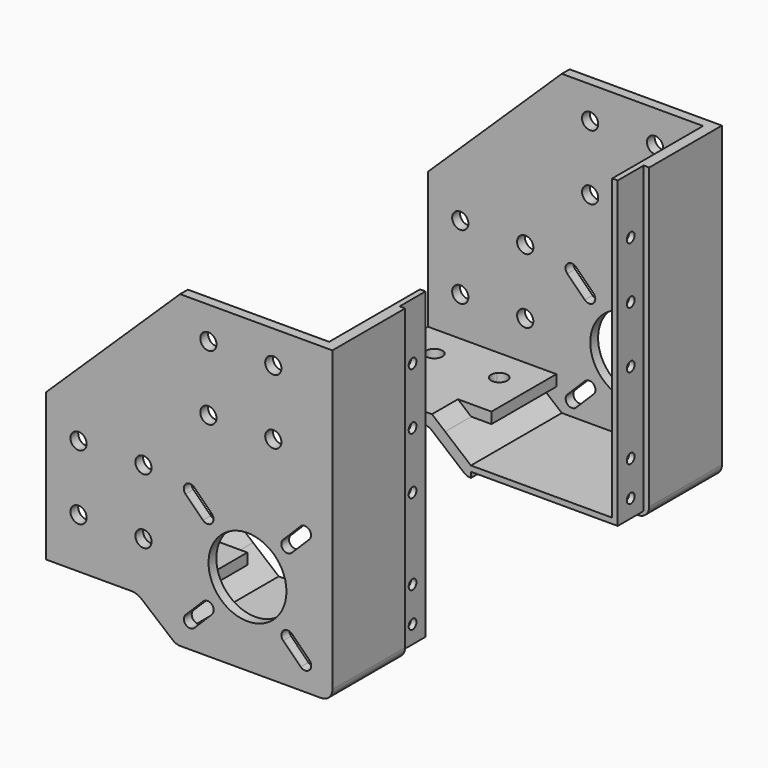
from build123d import *

# Parameters (mm, degrees)
F3_R         = 2.5
F3_R_2       = 12
F5_DEPTH     = 3
F6_DEPTH     = 28
F7_R         = 2.5
F8_DEPTH     = 12.5
F9_DEPTH     = 207
F11_DEPTH    = 10
F12_R        = 1.5
F13_DEPTH    = 1.7
F14_T1_DEPTH = 44.1548490014
F14_T3_DEPTH = 45
F15_R        = 5


# Not quite as in the source:
# - a fillet or chamfer that OpenCascade refuses, or shapes differently, is made with other operations: its cross-section is extruded or revolved along the edge and cut away or added
# - an extrude ends at something that could not be found from the text; its depth is read off the source's solid


with BuildPart() as f5:
    # F3 (on offset) → F5 (new body)
    with BuildSketch(Plane.XZ.offset(75)):
        Polygon((22.8, -22), (22.8, 22), (-11.1900709997, 22), (-20.7240998825, 30.0000001192), (-31.9999998808, 30.0000001192), (-61.9999998808, 30.0000001192), (-61.9999998808, -9.9999998808), (-61.9999998808, -11.9999998808), (-32.7240997633, -11.9999998808), (-20.7240998825, -22), align=None)
        with Locations((-51.9999998808, 1.192e-07)):
            Circle(F3_R, mode=Mode.SUBTRACT)
        with Locations((-31.9999998808, 1.192e-07)):
            Circle(F3_R, mode=Mode.SUBTRACT)
        with Locations((-51.9999998808, 20.0000001192)):
            Circle(F3_R, mode=Mode.SUBTRACT)
        with Locations((-31.9999998808, 20.0000001192)):
            Circle(F3_R, mode=Mode.SUBTRACT)
        with BuildLine():
            Line((-10.9146282961, -13.6954990502), (-16.2886398331, -19.0695105872))
            ThreePointArc((-16.2886398331, -19.0695105872), (-18.9756456016, -19.0695105872), (-18.9756456016, -16.3825048187))
            Line((-18.9756456016, -16.3825048187), (-13.6016340646, -11.0084932817))
            ThreePointArc((-13.6016340646, -11.0084932817), (-10.9146282961, -11.0084932817), (-10.9146282961, -13.6954990502))
        make_face(mode=Mode.SUBTRACT)
        with Locations((0.0469324928, 0.0079305583)):
            Circle(F3_R_2, mode=Mode.SUBTRACT)
        with BuildLine():
            Line((13.7503621014, -10.9536302305), (19.1243736384, -16.3276417676))
            ThreePointArc((19.1243736384, -16.3276417676), (19.1243736384, -19.0146475361), (16.4373678699, -19.0146475361))
            Line((16.4373678699, -19.0146475361), (11.0633563329, -13.6406359991))
            ThreePointArc((11.0633563329, -13.6406359991), (11.0633563329, -10.9536302305), (13.7503621014, -10.9536302305))
        make_face(mode=Mode.SUBTRACT)
        with BuildLine():
            ThreePointArc((-10.9694913472, 13.6564971157), (-10.9694913472, 10.9694913472), (-13.6564971157, 10.9694913472))
            Line((-13.6564971157, 10.9694913472), (-19.0305086528, 16.3435028843))
            ThreePointArc((-19.0305086528, 16.3435028843), (-19.0305086528, 19.0305086528), (-16.3435028843, 19.0305086528))
            Line((-16.3435028843, 19.0305086528), (-10.9694913472, 13.6564971157))
        make_face(mode=Mode.SUBTRACT)
        with BuildLine():
            Line((11.0084932817, 13.7113601669), (16.3825048187, 19.0853717039))
            ThreePointArc((16.3825048187, 19.0853717039), (19.0695105872, 19.0853717039), (19.0695105872, 16.3983659354))
            Line((19.0695105872, 16.3983659354), (13.6954990502, 11.0243543984))
            ThreePointArc((13.6954990502, 11.0243543984), (11.0084932817, 11.0243543984), (11.0084932817, 13.7113601669))
        make_face(mode=Mode.SUBTRACT)
        Polygon((-11.1900709997, 22), (22.8, 22), (22.8, 70.0000001192), (-20.7240998825, 70.0000001192), (-61.9999998808, 30.0000001192), (-31.9999998808, 30.0000001192), (-20.7240998825, 30.0000001192), align=None)
        with Locations((-11.9999998808, 40.0000001192)):
            Circle(F3_R, mode=Mode.SUBTRACT)
        with Locations((8.0000001192, 40.0000001192)):
            Circle(F3_R, mode=Mode.SUBTRACT)
        with Locations((-11.9999998808, 60.0000001192)):
            Circle(F3_R, mode=Mode.SUBTRACT)
        with Locations((8.0000001192, 60.0000001192)):
            Circle(F3_R, mode=Mode.SUBTRACT)
    extrude(amount=-F5_DEPTH)

    # F4 (on offset) → F6 (join)
    with BuildSketch(Plane.XZ.offset(75)):
        Polygon((-32.7240997633, -11.9999998808), (-61.9999998808, -11.9999998808), (-61.9999998808, -15.3999998808), (-33.9550695636, -15.3999998808), (-21.9550696828, -25.4), (22.8, -25.4), (22.8, -22), (-20.7240998825, -22), (-28.6440998525, -15.3999998808), align=None)
        Polygon((-22.4, -11.9999998808), (-32.7240997633, -11.9999998808), (-28.6440998525, -15.3999998808), (-22.4, -15.3999998808), align=None)
        Polygon((22.8, 22), (22.8, -22), (22.8, -25.4), (26.2, -25.4), (26.2, 22), (26.2, 70.0000001192), (22.8, 70.0000001192), align=None)
    extrude(amount=-F6_DEPTH)

    # F7 (on face) → F8 (cut, symmetric)
    with BuildSketch(Plane(origin=(0, 0, -15.3999998808), x_dir=(1, 0, 0), z_dir=(0, 0, -1))):
        with BuildLine():
            Line((-33.9550695636, 60.4418913596), (-33.9550695636, 63.5581086404))
            ThreePointArc((-33.9550695636, 63.5581086404), (-34.4999998808, 62), (-33.9550695636, 60.4418913596))
        make_face()
        with BuildLine():
            ThreePointArc((-33.9550695636, 60.4418913596), (-31.1746739473, 59.6401616361), (-29.4999998808, 62))
            ThreePointArc((-29.4999998808, 62), (-31.1746739473, 64.3598383639), (-33.9550695636, 63.5581086404))
            Line((-33.9550695636, 63.5581086404), (-33.9550695636, 60.4418913596))
        make_face()
        with Locations((-51.9999998808, 62)):
            Circle(F7_R)
    extrude(amount=F8_DEPTH, both=True, mode=Mode.SUBTRACT)

    # F7 (on face) → F9 (cut, through all)
    with BuildSketch(Plane(origin=(0, 0, -15.3999998808), x_dir=(1, 0, 0), z_dir=(0, 0, -1))):
        with BuildLine():
            ThreePointArc((-33.9550695636, 60.4418913596), (-34.4999998808, 62), (-33.9550695636, 63.5581086404))
            Line((-33.9550695636, 63.5581086404), (-33.9550695636, 66.0531102299))
            ThreePointArc((-33.9550695636, 66.0531102299), (-36.4999998808, 62), (-33.9550695636, 57.9468897701))
            Line((-33.9550695636, 57.9468897701), (-33.9550695636, 60.4418913596))
        make_face()
        with BuildLine():
            ThreePointArc((-33.9550695636, 63.5581086404), (-31.1746739473, 64.3598383639), (-29.4999998808, 62))
            ThreePointArc((-29.4999998808, 62), (-31.1746739473, 59.6401616361), (-33.9550695636, 60.4418913596))
            Line((-33.9550695636, 60.4418913596), (-33.9550695636, 57.9468897701))
            ThreePointArc((-33.9550695636, 57.9468897701), (-29.6070742209, 58.1889756251), (-27.4999998808, 62))
            ThreePointArc((-27.4999998808, 62), (-29.6070742209, 65.8110243749), (-33.9550695636, 66.0531102299))
            Line((-33.9550695636, 66.0531102299), (-33.9550695636, 63.5581086404))
        make_face()
        with BuildLine():
            Line((-33.9550695636, 60.4418913596), (-33.9550695636, 63.5581086404))
            ThreePointArc((-33.9550695636, 63.5581086404), (-34.4999998808, 62), (-33.9550695636, 60.4418913596))
        make_face()
        with BuildLine():
            ThreePointArc((-33.9550695636, 60.4418913596), (-31.1746739473, 59.6401616361), (-29.4999998808, 62))
            ThreePointArc((-29.4999998808, 62), (-31.1746739473, 64.3598383639), (-33.9550695636, 63.5581086404))
            Line((-33.9550695636, 63.5581086404), (-33.9550695636, 60.4418913596))
        make_face()
    extrude(amount=F9_DEPTH, mode=Mode.SUBTRACT)

    # F10 (on face) → F11 (join)
    with BuildSketch(Plane(origin=(0, -47, 0), x_dir=(-1, 0, 0), z_dir=(0, 1, 0))):
        Polygon((20.7240998825, -22), (-22.8, -22), (-22.8, 70.0000001192), (-24.5, 70.0000001192), (-24.5, -23.7), (20.7240998825, -23.7), (20.7240998825, -25.4), (21.9550696828, -25.4), (33.9550695636, -15.3999998808), (61.9999998808, -15.3999998808), (61.9999998808, -11.9999998808), (32.7240997633, -11.9999998808), (28.6440998525, -15.3999998808), align=None)
    extrude(amount=F11_DEPTH)

    # F12 (on face) → F13 (cut, through all)
    with BuildSketch(Plane.YZ.offset(24.5)):
        with Locations((-42, -7.4259215035)):
            Circle(F12_R)
        with Locations((-42, -18.2226523757)):
            Circle(F12_R)
        with Locations((-42, 52.5000000894)):
            Circle(F12_R)
        with Locations((-42, 35.0000000596)):
            Circle(F12_R)
        with Locations((-42, 17.5000000298)):
            Circle(F12_R)
    extrude(amount=-F13_DEPTH, mode=Mode.SUBTRACT)

    # F14: fillet of radius 3.4 on 2 edges, made by hand

    # F14_s2 → F14_t1 (cut)
    with BuildSketch(Plane.XZ.offset(33.9225754993)):
        with BuildLine():
            ThreePointArc((-22.9007268695, -24.6119523272), (-21.8815457965, -25.1969233579), (-20.7240998825, -25.4))
            Line((-20.7240998825, -25.4), (-21.9550696828, -25.4))
            Line((-21.9550696828, -25.4), (-22.9007268695, -24.6119523272))
        make_face()
    extrude(amount=F14_T1_DEPTH, mode=Mode.SUBTRACT)

    # F14_s4 → F14_t3 (cut)
    with BuildSketch(Plane.XZ.offset(38.5)):
        with BuildLine():
            ThreePointArc((22.8, -25.4), (25.204163056, -24.404163056), (26.2, -22))
            Line((26.2, -22), (26.2, -25.4))
            Line((26.2, -25.4), (22.8, -25.4))
        make_face()
    extrude(amount=F14_T3_DEPTH, mode=Mode.SUBTRACT)

    # F15
    f15_edges = [f5.edges().sort_by_distance(p)[0] for p in [
        (-33.95507, -70.526555, -15.4),
        (-33.95507, -47.473445, -15.4),
    ]]
    fillet(f15_edges, radius=F15_R)


with BuildPart() as f16_1:
    # F16: instance of F5
    add(f5.part.mirror(Plane.XZ))


solid = Compound([f5.part, f16_1.part])
